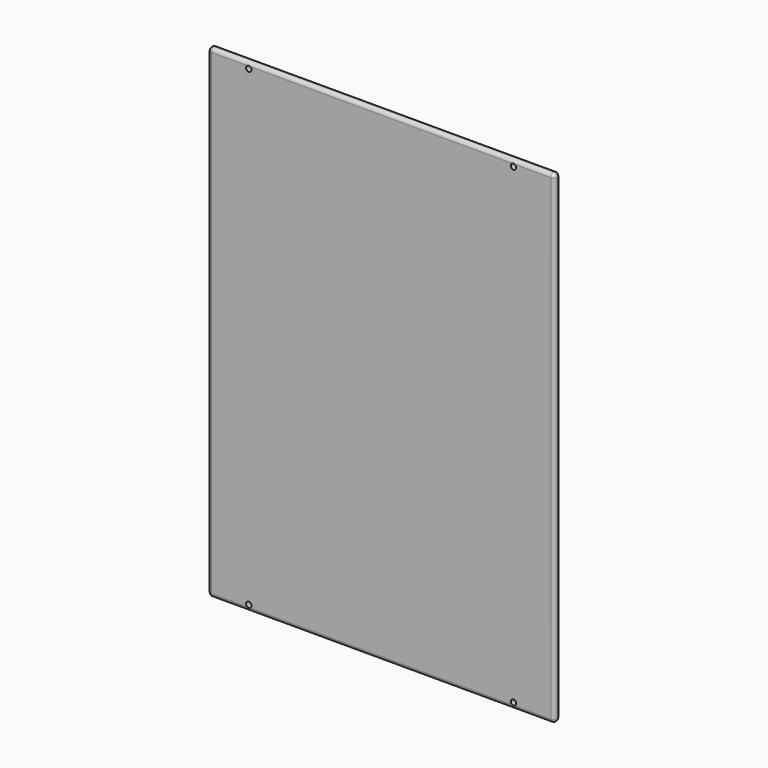
from build123d import *

# Parameters (mm, degrees)
F0_W         = 457.2
F0_H         = 638.175
F1_DEPTH     = 9.525
F3_D         = 7.14375
F4_T1_DEPTH  = 628.6502
F4_T3_DEPTH  = 447.6752
F4_T5_DEPTH  = 0.0002
F4_S9_W      = 4.85775
F4_S9_H      = 4.85775
F4_T10_DEPTH = 4.85775
F4_S15_W     = 4.85775
F4_S15_H     = 4.85775
F4_T16_DEPTH = 4.85775
F4_S21_W     = 4.85775
F4_S21_H     = 4.85775
F4_T22_DEPTH = 4.85775
F4_S27_W     = 4.85775
F4_S27_H     = 4.85775
F4_T28_DEPTH = 4.85775
F4_S33_W     = 4.85775
F4_S33_H     = 4.85775
F4_T34_DEPTH = 4.85775
F4_S39_W     = 4.85775
F4_S39_H     = 4.85775
F4_T40_DEPTH = 4.85775
F4_S45_W     = 4.85775
F4_S45_H     = 4.85775
F4_T46_DEPTH = 4.85775
F4_S51_W     = 4.85775
F4_S51_H     = 4.85775
F4_T52_DEPTH = 4.85775


# Not quite as in the source:
# - a fillet or chamfer that OpenCascade refuses, or shapes differently, is made with other operations: its cross-section is extruded or revolved along the edge and cut away or added


with BuildPart() as f1:
    # F0 (on Front) → F1 (new body)
    with BuildSketch(Plane.XZ):
        Rectangle(F0_W, F0_H)
    extrude(amount=F1_DEPTH)

    # F3 (through all)
    with Locations(Plane.XZ.offset(9.525)):
        with Locations((-174.625, 311.15), (174.625, 311.15), (-174.625, -311.15), (174.625, -311.15)):
            Hole(F3_D / 2)

    # F4: fillet of radius 4.7625 on 12 edges, made by hand

    # F4_s2 → F4_t1 (cut)
    with BuildSketch(Plane.XY.offset(-314.3251)):
        with BuildLine():
            ThreePointArc((-228.6001, -4.7626), (-227.2051960454, -8.1301960454), (-223.8376, -9.5251))
            Line((-223.8376, -9.5251), (-223.8376, -9.62035))
            ThreePointArc((-223.8376, -9.62035), (-226.2188, -9.62025), (-228.6, -9.62025))
            Line((-228.6, -9.62025), (-228.69525, -9.525))
            ThreePointArc((-228.69525, -9.525), (-228.69525, -7.1438), (-228.69535, -4.7626))
            Line((-228.69535, -4.7626), (-228.6001, -4.7626))
        make_face()
        with BuildLine():
            ThreePointArc((228.6001, -4.7626), (227.2051960454, -8.1301960454), (223.8376, -9.5251))
            Line((223.8376, -9.5251), (223.8376, -9.62035))
            ThreePointArc((223.8376, -9.62035), (226.2188, -9.62025), (228.6, -9.62025))
            Line((228.6, -9.62025), (228.69525, -9.525))
            ThreePointArc((228.69525, -9.525), (228.69525, -7.1438), (228.69535, -4.7626))
            Line((228.69535, -4.7626), (228.6001, -4.7626))
        make_face()
        with BuildLine():
            ThreePointArc((228.6001, -4.7624), (227.2051960454, -1.3948039546), (223.8376, 0.0001))
            Line((223.8376, 0.0001), (223.8376, 0.09535))
            ThreePointArc((223.8376, 0.09535), (226.2188, 0.09525), (228.6, 0.09525))
            Line((228.6, 0.09525), (228.69525, 0))
            ThreePointArc((228.69525, 0), (228.69525, -2.3812), (228.69535, -4.7624))
            Line((228.69535, -4.7624), (228.6001, -4.7624))
        make_face()
        with BuildLine():
            ThreePointArc((-228.6001, -4.7624), (-227.2051960454, -1.3948039546), (-223.8376, 0.0001))
            Line((-223.8376, 0.0001), (-223.8376, 0.09535))
            ThreePointArc((-223.8376, 0.09535), (-226.2188, 0.09525), (-228.6, 0.09525))
            Line((-228.6, 0.09525), (-228.69525, 0))
            ThreePointArc((-228.69525, 0), (-228.69525, -2.3812), (-228.69535, -4.7624))
            Line((-228.69535, -4.7624), (-228.6001, -4.7624))
        make_face()
    extrude(amount=F4_T1_DEPTH, mode=Mode.SUBTRACT)

    # F4_s4 → F4_t3 (cut)
    with BuildSketch(Plane.YZ.offset(-223.8376)):
        with BuildLine():
            ThreePointArc((-4.7626, -319.0876), (-8.1301960454, -317.6926960454), (-9.5251, -314.3251))
            Line((-9.5251, -314.3251), (-9.62035, -314.3251))
            ThreePointArc((-9.62035, -314.3251), (-9.62025, -316.7063), (-9.62025, -319.0875))
            Line((-9.62025, -319.0875), (-9.525, -319.18275))
            ThreePointArc((-9.525, -319.18275), (-7.1438, -319.18275), (-4.7626, -319.18285))
            Line((-4.7626, -319.18285), (-4.7626, -319.0876))
        make_face()
        with BuildLine():
            ThreePointArc((-9.5251, 314.3251), (-8.1301960454, 317.6926960454), (-4.7626, 319.0876))
            Line((-4.7626, 319.0876), (-4.7626, 319.18285))
            ThreePointArc((-4.7626, 319.18285), (-7.1438, 319.18275), (-9.525, 319.18275))
            Line((-9.525, 319.18275), (-9.62025, 319.0875))
            ThreePointArc((-9.62025, 319.0875), (-9.62025, 316.7063), (-9.62035, 314.3251))
            Line((-9.62035, 314.3251), (-9.5251, 314.3251))
        make_face()
        with BuildLine():
            ThreePointArc((0.0001, 314.3251), (-1.3948039546, 317.6926960454), (-4.7624, 319.0876))
            Line((-4.7624, 319.0876), (-4.7624, 319.18285))
            ThreePointArc((-4.7624, 319.18285), (-2.3812, 319.18275), (0, 319.18275))
            Line((0, 319.18275), (0.09525, 319.0875))
            ThreePointArc((0.09525, 319.0875), (0.09525, 316.7063), (0.09535, 314.3251))
            Line((0.09535, 314.3251), (0.0001, 314.3251))
        make_face()
        with BuildLine():
            ThreePointArc((-4.7624, -319.0876), (-1.3948039546, -317.6926960454), (0.0001, -314.3251))
            Line((0.0001, -314.3251), (0.09535, -314.3251))
            ThreePointArc((0.09535, -314.3251), (0.09525, -316.7063), (0.09525, -319.0875))
            Line((0.09525, -319.0875), (0, -319.18275))
            ThreePointArc((0, -319.18275), (-2.3812, -319.18275), (-4.7624, -319.18285))
            Line((-4.7624, -319.18285), (-4.7624, -319.0876))
        make_face()
    extrude(amount=F4_T3_DEPTH, mode=Mode.SUBTRACT)

    # F4_s6 → F4_t5 (cut)
    with BuildSketch(Plane.XZ.offset(4.7624)):
        with BuildLine():
            ThreePointArc((-223.8376, -319.0876), (-227.2051960454, -317.6926960454), (-228.6001, -314.3251))
            Line((-228.6001, -314.3251), (-228.69535, -314.3251))
            ThreePointArc((-228.69535, -314.3251), (-228.69525, -316.7063), (-228.69525, -319.0875))
            Line((-228.69525, -319.0875), (-228.6, -319.18275))
            ThreePointArc((-228.6, -319.18275), (-226.2188, -319.18275), (-223.8376, -319.18285))
            Line((-223.8376, -319.18285), (-223.8376, -319.0876))
        make_face()
        with BuildLine():
            ThreePointArc((223.8376, -319.0876), (227.2051960454, -317.6926960454), (228.6001, -314.3251))
            Line((228.6001, -314.3251), (228.69535, -314.3251))
            ThreePointArc((228.69535, -314.3251), (228.69525, -316.7063), (228.69525, -319.0875))
            Line((228.69525, -319.0875), (228.6, -319.18275))
            ThreePointArc((228.6, -319.18275), (226.2188, -319.18275), (223.8376, -319.18285))
            Line((223.8376, -319.18285), (223.8376, -319.0876))
        make_face()
        with BuildLine():
            ThreePointArc((228.6001, 314.3251), (227.2051960454, 317.6926960454), (223.8376, 319.0876))
            Line((223.8376, 319.0876), (223.8376, 319.18285))
            ThreePointArc((223.8376, 319.18285), (226.2188, 319.18275), (228.6, 319.18275))
            Line((228.6, 319.18275), (228.69525, 319.0875))
            ThreePointArc((228.69525, 319.0875), (228.69525, 316.7063), (228.69535, 314.3251))
            Line((228.69535, 314.3251), (228.6001, 314.3251))
        make_face()
        with BuildLine():
            ThreePointArc((-228.6001, 314.3251), (-227.2051960454, 317.6926960454), (-223.8376, 319.0876))
            Line((-223.8376, 319.0876), (-223.8376, 319.18285))
            ThreePointArc((-223.8376, 319.18285), (-226.2188, 319.18275), (-228.6, 319.18275))
            Line((-228.6, 319.18275), (-228.69525, 319.0875))
            ThreePointArc((-228.69525, 319.0875), (-228.69525, 316.7063), (-228.69535, 314.3251))
            Line((-228.69535, 314.3251), (-228.6001, 314.3251))
        make_face()
    extrude(amount=F4_T5_DEPTH, mode=Mode.SUBTRACT)


with BuildPart() as f4_tool8:
    # F4_s9 → F4_t10 (new body)
    with BuildSketch(Plane.YZ.offset(-223.8376)):
        with Locations((-7.191475, 316.753975)):
            Rectangle(F4_S9_W, F4_S9_H)
    extrude(amount=-F4_T10_DEPTH)

    # F4_s11 → F4_t12 (revolve, cut)
    with BuildSketch(Plane(origin=(-223.8376, -4.7626, 314.3251), x_dir=(0, 0.7071067812, -0.7071067812), z_dir=(0, 0.7071067812, 0.7071067812))):
        with BuildLine():
            ThreePointArc((0, -4.7625), (4.7625, 0), (0, 4.7625))
            Line((0, 4.7625), (0, -4.7625))
        make_face()
    revolve(axis=Axis((-223.8376, -4.7626, 314.3251), (-1, 0, 0)), mode=Mode.SUBTRACT)


with BuildPart() as f1_1:
    add(f1.part)

    # F4_t7: cut F4_tool8
    add(f4_tool8.part, mode=Mode.SUBTRACT)


with BuildPart() as f4_tool14:
    # F4_s15 → F4_t16 (new body)
    with BuildSketch(Plane.XY.offset(-314.3251)):
        with Locations((-226.266475, -7.191475)):
            Rectangle(F4_S15_W, F4_S15_H)
    extrude(amount=-F4_T16_DEPTH)

    # F4_s17 → F4_t18 (revolve, cut)
    with BuildSketch(Plane(origin=(-223.8376, -4.7626, -314.3251), x_dir=(0.7071067812, 0.7071067812, 0), z_dir=(-0.7071067812, 0.7071067812, 0))):
        with BuildLine():
            ThreePointArc((0, -4.7625), (4.7625, 0), (0, 4.7625))
            Line((0, 4.7625), (0, -4.7625))
        make_face()
    revolve(axis=Axis((-223.8376, -4.7626, -314.3251), (0, 0, -1)), mode=Mode.SUBTRACT)


with BuildPart() as f1_2:
    add(f1_1.part)

    # F4_t13: cut F4_tool14
    add(f4_tool14.part, mode=Mode.SUBTRACT)


with BuildPart() as f4_tool20:
    # F4_s21 → F4_t22 (new body)
    with BuildSketch(Plane.XY.offset(-314.3251)):
        with Locations((226.266475, -7.191475)):
            Rectangle(F4_S21_W, F4_S21_H)
    extrude(amount=-F4_T22_DEPTH)

    # F4_s23 → F4_t24 (revolve, cut)
    with BuildSketch(Plane(origin=(223.8376, -4.7626, -314.3251), x_dir=(-0.7071067812, 0.7071067812, 0), z_dir=(-0.7071067812, -0.7071067812, 0))):
        with BuildLine():
            ThreePointArc((0, -4.7625), (4.7625, 0), (0, 4.7625))
            Line((0, 4.7625), (0, -4.7625))
        make_face()
    revolve(axis=Axis((223.8376, -4.7626, -314.3251), (0, 0, -1)), mode=Mode.SUBTRACT)


with BuildPart() as f1_3:
    add(f1_2.part)

    # F4_t19: cut F4_tool20
    add(f4_tool20.part, mode=Mode.SUBTRACT)


with BuildPart() as f4_tool26:
    # F4_s27 → F4_t28 (new body)
    with BuildSketch(Plane.YZ.offset(223.8376)):
        with Locations((-7.191475, 316.753975)):
            Rectangle(F4_S27_W, F4_S27_H)
    extrude(amount=F4_T28_DEPTH)

    # F4_s29 → F4_t30 (revolve, cut)
    with BuildSketch(Plane(origin=(223.8376, -4.7626, 314.3251), x_dir=(0, 0.7071067812, -0.7071067812), z_dir=(0, -0.7071067812, -0.7071067812))):
        with BuildLine():
            ThreePointArc((0, -4.7625), (4.7625, 0), (0, 4.7625))
            Line((0, 4.7625), (0, -4.7625))
        make_face()
    revolve(axis=Axis((223.8376, -4.7626, 314.3251), (1, 0, 0)), mode=Mode.SUBTRACT)


with BuildPart() as f1_4:
    add(f1_3.part)

    # F4_t25: cut F4_tool26
    add(f4_tool26.part, mode=Mode.SUBTRACT)


with BuildPart() as f4_tool32:
    # F4_s33 → F4_t34 (new body)
    with BuildSketch(Plane.XY.offset(-314.3251)):
        with Locations((226.266475, -2.333525)):
            Rectangle(F4_S33_W, F4_S33_H)
    extrude(amount=-F4_T34_DEPTH)

    # F4_s35 → F4_t36 (revolve, cut)
    with BuildSketch(Plane(origin=(223.8376, -4.7624, -314.3251), x_dir=(-0.7071067812, -0.7071067812, 0), z_dir=(0.7071067812, -0.7071067812, 0))):
        with BuildLine():
            ThreePointArc((0, -4.7625), (4.7625, 0), (0, 4.7625))
            Line((0, 4.7625), (0, -4.7625))
        make_face()
    revolve(axis=Axis((223.8376, -4.7624, -314.3251), (0, 0, -1)), mode=Mode.SUBTRACT)


with BuildPart() as f1_5:
    add(f1_4.part)

    # F4_t31: cut F4_tool32
    add(f4_tool32.part, mode=Mode.SUBTRACT)


with BuildPart() as f4_tool38:
    # F4_s39 → F4_t40 (new body)
    with BuildSketch(Plane.YZ.offset(223.8376)):
        with Locations((-2.333525, 316.753975)):
            Rectangle(F4_S39_W, F4_S39_H)
    extrude(amount=F4_T40_DEPTH)

    # F4_s41 → F4_t42 (revolve, cut)
    with BuildSketch(Plane(origin=(223.8376, -4.7624, 314.3251), x_dir=(0, -0.7071067812, -0.7071067812), z_dir=(0, -0.7071067812, 0.7071067812))):
        with BuildLine():
            ThreePointArc((0, -4.7625), (4.7625, 0), (0, 4.7625))
            Line((0, 4.7625), (0, -4.7625))
        make_face()
    revolve(axis=Axis((223.8376, -4.7624, 314.3251), (1, 0, 0)), mode=Mode.SUBTRACT)


with BuildPart() as f1_6:
    add(f1_5.part)

    # F4_t37: cut F4_tool38
    add(f4_tool38.part, mode=Mode.SUBTRACT)


with BuildPart() as f4_tool44:
    # F4_s45 → F4_t46 (new body)
    with BuildSketch(Plane.YZ.offset(-223.8376)):
        with Locations((-2.333525, 316.753975)):
            Rectangle(F4_S45_W, F4_S45_H)
    extrude(amount=-F4_T46_DEPTH)

    # F4_s47 → F4_t48 (revolve, cut)
    with BuildSketch(Plane(origin=(-223.8376, -4.7624, 314.3251), x_dir=(0, -0.7071067812, -0.7071067812), z_dir=(0, 0.7071067812, -0.7071067812))):
        with BuildLine():
            ThreePointArc((0, -4.7625), (4.7625, 0), (0, 4.7625))
            Line((0, 4.7625), (0, -4.7625))
        make_face()
    revolve(axis=Axis((-223.8376, -4.7624, 314.3251), (-1, 0, 0)), mode=Mode.SUBTRACT)


with BuildPart() as f1_7:
    add(f1_6.part)

    # F4_t43: cut F4_tool44
    add(f4_tool44.part, mode=Mode.SUBTRACT)


with BuildPart() as f4_tool50:
    # F4_s51 → F4_t52 (new body)
    with BuildSketch(Plane.XY.offset(-314.3251)):
        with Locations((-226.266475, -2.333525)):
            Rectangle(F4_S51_W, F4_S51_H)
    extrude(amount=-F4_T52_DEPTH)

    # F4_s53 → F4_t54 (revolve, cut)
    with BuildSketch(Plane(origin=(-223.8376, -4.7624, -314.3251), x_dir=(0.7071067812, -0.7071067812, 0), z_dir=(0.7071067812, 0.7071067812, 0))):
        with BuildLine():
            ThreePointArc((0, -4.7625), (4.7625, 0), (0, 4.7625))
            Line((0, 4.7625), (0, -4.7625))
        make_face()
    revolve(axis=Axis((-223.8376, -4.7624, -314.3251), (0, 0, -1)), mode=Mode.SUBTRACT)


with BuildPart() as f1_8:
    add(f1_7.part)

    # F4_t49: cut F4_tool50
    add(f4_tool50.part, mode=Mode.SUBTRACT)


solid = f1_8.part
